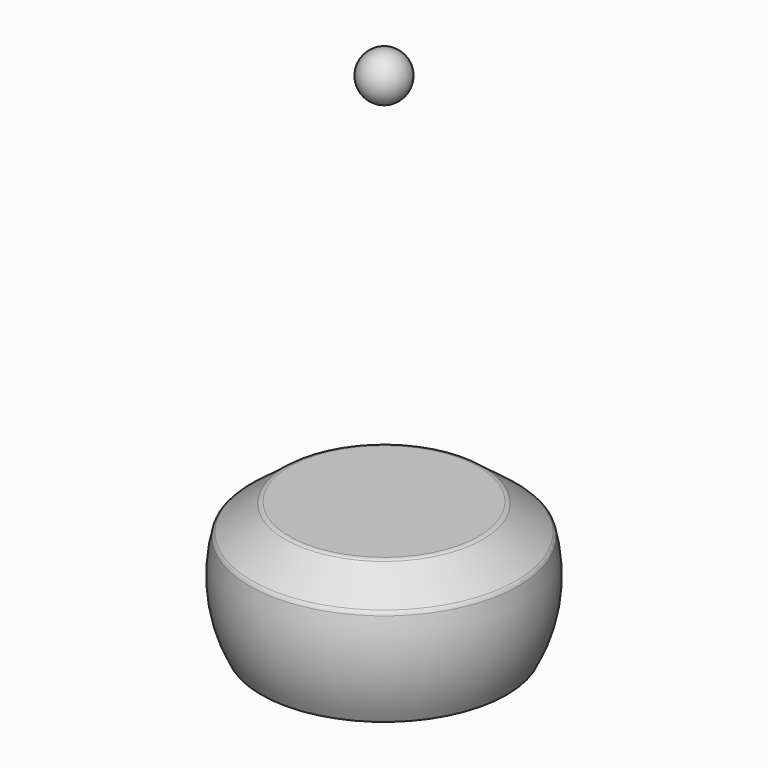
from build123d import *

# Parameters (mm, degrees)
F4_R = 1.5
F5_R = 1.5


# Not quite as in the source:
# - a fillet or chamfer that OpenCascade refuses, or shapes differently, is made with other operations: its cross-section is extruded or revolved along the edge and cut away or added
# - the program builds the solid bodies; features that only make, move or delete a surface that nothing else refers to are left out


with BuildPart() as f2:
    # F0 (on Front) → F2 (revolve)
    with BuildSketch(Plane.XZ):
        with BuildLine():
            Line((0, 14.0623611104), (0, -14.0623611104))
            Line((0, -14.0623611104), (26.5, -14.0623611104))
            ThreePointArc((26.5, -14.0623611104), (30, 0), (26.5, 14.0623611104))
            Line((26.5, 14.0623611104), (0, 14.0623611104))
        make_face()
    revolve(axis=Axis((0, 0, -0.4438906908), (0, 0, -1)))

    # F3: chamfer of 5 on 1 edges, made by hand

    # F3_s1 → F3_t2 (revolve, cut)
    with BuildSketch(Plane.XZ):
        with BuildLine():
            Line((29.0858230111, 7.8312895768), (20.7514586352, 14.1835977215))
            Line((20.7514586352, 14.1835977215), (20.7514586352, 14.2835977215))
            ThreePointArc((20.7514586352, 14.2835977215), (23.6257293176, 14.1623611104), (26.5, 14.1623611104))
            Line((26.5, 14.1623611104), (26.5883333333, 14.1092356475))
            ThreePointArc((26.5883333333, 14.1092356475), (28.005944571, 11.0307329169), (29.1822455377, 7.8577979974))
            Line((29.1822455377, 7.8577979974), (29.0858230111, 7.8312895768))
        make_face()
    revolve(axis=Axis((0, 0, 14.0623611104), (0, 0, -1)), mode=Mode.SUBTRACT)

    # F4
    f4_edges = [f2.edges().sort_by_distance(p)[0] for p in [
        (-20.910524, 0, 14.062361),
    ]]
    fillet(f4_edges, radius=F4_R)

    # F5
    f5_edges = [f2.edges().sort_by_distance(p)[0] for p in [
        (-28.926758, 0, 7.952526),
    ]]
    fillet(f5_edges, radius=F5_R)


with BuildPart() as f7:
    # F0 (on Front) → F7 (revolve)
    with BuildSketch(Plane.XZ):
        with BuildLine():
            ThreePointArc((0, 90), (5, 95), (0, 100))
            Line((0, 100), (0, 90))
        make_face()
    revolve(axis=Axis((0, 0, -0.4438906908), (0, 0, -1)))


solid = Compound([f2.part, f7.part])
